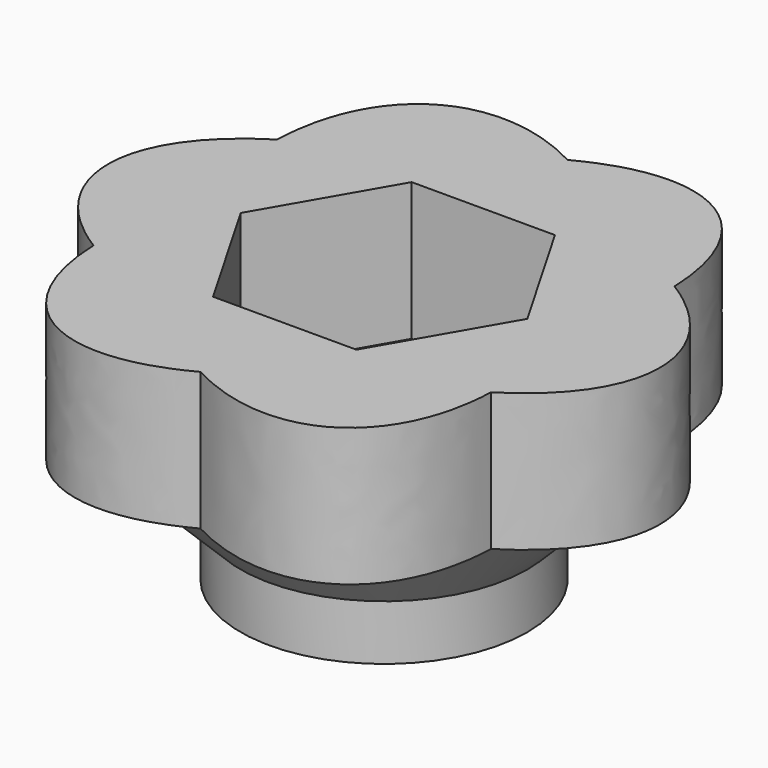
from build123d import *

# Parameters (mm, degrees)
F0_R     = 6.604
F0_R_2   = 3.175
F1_DEPTH = 2.54
F2_R     = 10.414
F2_R_2   = 6.604
F2_R_3   = 3.175
F3_DEPTH = 3.81
F4_SIZE  = 3.80999
F6_DEPTH = 6.35


# Not quite as in the source:
# - a fillet or chamfer is up to 0.001 mm smaller than in the source, because OpenCascade refuses the exact size


with BuildPart() as f1:
    # F0 (on Top) → F1 (new body)
    with BuildSketch(Plane.XY):
        Circle(F0_R)
        Circle(F0_R_2, mode=Mode.SUBTRACT)
    extrude(amount=F1_DEPTH)

    # F2 (on face) → F3 (join)
    with BuildSketch(Plane.XY.offset(2.54)):
        Circle(F2_R)
        Circle(F2_R_2, mode=Mode.SUBTRACT)
        Circle(F2_R_2)
        Circle(F2_R_3, mode=Mode.SUBTRACT)
    extrude(amount=F3_DEPTH)

    # F4 (size 3.81 in the source; OpenCascade refuses exactly that, so slightly less here)
    f4_edges = [f1.edges().sort_by_distance(p)[0] for p in [
        (-10.414, 0, 2.54),
    ]]
    chamfer(f4_edges, length=F4_SIZE)

    # F5 (on face) → F6 (join)
    with BuildSketch(Plane.XY.offset(6.35)):
        with BuildLine():
            add(Edge.make_bspline(
                [(0, -10.5673162871), (8.8130461977, -15.2646437839), (9.1515643544, -5.2836581435)],
                knots=[2.3754047296, 2.3754047296, 2.3754047296, 3.9077805776, 3.9077805776, 3.9077805776], degree=2, weights=[1, 0.7205591673, 1]))
            add(Edge.make_bspline(
                [(9.1515643544, -5.2836581435), (17.6260923954, 0), (9.1515643544, 5.2836581435)],
                knots=[5.5169973832, 5.5169973832, 5.5169973832, 7.0493732312, 7.0493732312, 7.0493732312], degree=2, weights=[1, 0.7205591673, 1]))
            add(Edge.make_bspline(
                [(9.1515643544, 5.2836581435), (8.8130461977, 15.2646437839), (0, 10.5673162871)],
                knots=[2.3754047296, 2.3754047296, 2.3754047296, 3.9077805776, 3.9077805776, 3.9077805776], degree=2, weights=[1, 0.7205591673, 1]))
            add(Edge.make_bspline(
                [(0, 10.5673162871), (-8.8130461977, 15.2646437839), (-9.1515643544, 5.2836581435)],
                knots=[5.5169973832, 5.5169973832, 5.5169973832, 7.0493732312, 7.0493732312, 7.0493732312], degree=2, weights=[1, 0.7205591673, 1]))
            add(Edge.make_bspline(
                [(-9.1515643544, 5.2836581435), (-17.6260923954, 0), (-9.1515643544, -5.2836581435)],
                knots=[2.3754047296, 2.3754047296, 2.3754047296, 3.9077805776, 3.9077805776, 3.9077805776], degree=2, weights=[1, 0.7205591673, 1]))
            add(Edge.make_bspline(
                [(-9.1515643544, -5.2836581435), (-8.8130461977, -15.2646437839), (0, -10.5673162871)],
                knots=[5.5169973832, 5.5169973832, 5.5169973832, 7.0493732312, 7.0493732312, 7.0493732312], degree=2, weights=[1, 0.7205591673, 1]))
        make_face()
        Polygon((-6.5991135768, 0), (-3.2995567884, 5.715), (3.2995567884, 5.715), (6.5991135768, 0), (3.2995567884, -5.715), (-3.2995567884, -5.715), align=None, mode=Mode.SUBTRACT)
    extrude(amount=F6_DEPTH)


solid = f1.part
